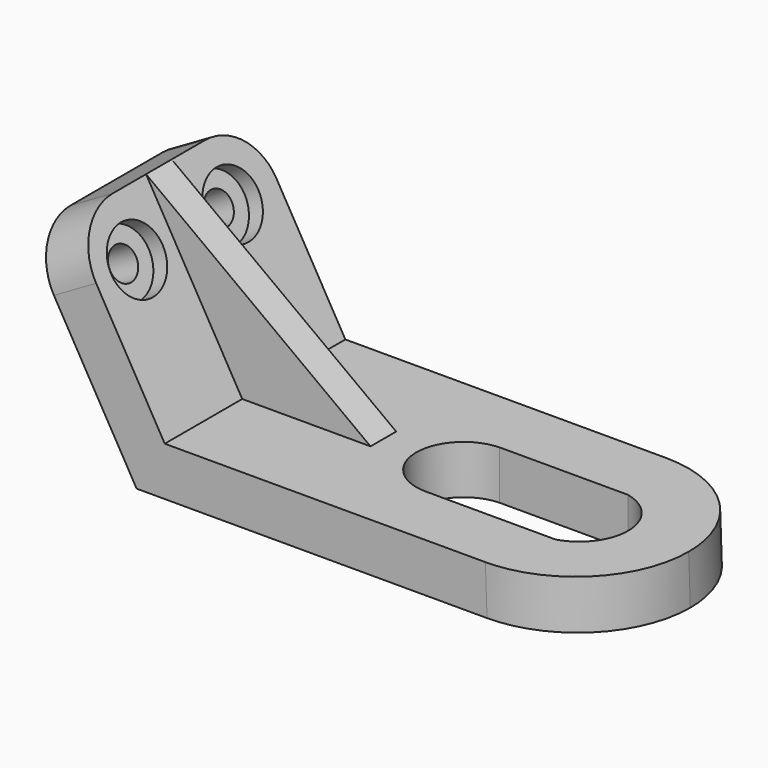
from build123d import *

# Parameters (mm, degrees)
F1_DEPTH  = 22.352
F2_DEPTH  = 3.175
F4_R      = 22.35199
F5_R      = 3.175
F6_DEPTH  = 25.4
F7_R      = 6.35
F7_R_2    = 3.175
F8_DEPTH  = 3.175
F9_R      = 10.922
F10_DEPTH = 25.4


# Not quite as in the source:
# - a fillet or chamfer is up to 0.001 mm smaller than in the source, because OpenCascade refuses the exact size


with BuildPart() as f1:
    # F0 (on Front) → F1 (new body, symmetric)
    with BuildSketch(Plane.XZ):
        Polygon((-3.9430456236, 0), (-29.3430456236, 0), (-48.3930456236, 32.9955678842), (-56.7519228209, 28.1695678842), (-34.9156304218, -9.652), (56.8391502193, -9.652), (56.5089543764, 0), align=None)
    extrude(amount=F1_DEPTH, both=True)

    # F0 (on Front) → F2 (join, symmetric)
    with BuildSketch(Plane.XZ):
        Polygon((-48.3930456236, 32.9955678842), (-29.3430456236, 0), (-3.9430456236, 0), align=None)
    extrude(amount=F2_DEPTH, both=True)

    # F4 (radius 22.352 in the source; OpenCascade refuses exactly that, so slightly less here)
    f4_edges = [f1.edges().sort_by_distance(p)[0] for p in [
        (56.674052, -22.352, -4.826),
        (56.674052, 22.352, -4.826),
    ]]
    fillet(f4_edges, radius=F4_R)

    # F5 (on face) → F6 (cut)
    with BuildSketch(Plane(origin=(-30.366161415, 0, -17.5319114672), x_dir=(0, -1, 0), z_dir=(-0.8660254038, 0, -0.5))):
        with Locations((-11.43, 41.8495228118)):
            Circle(F5_R)
        with Locations((12.2398376594, 41.8495228118)):
            Circle(F5_R)
    extrude(amount=-F6_DEPTH, mode=Mode.SUBTRACT)

    # F7 (on face) → F8 (cut)
    with BuildSketch(Plane(origin=(-22.0072842177, 0, -12.7059114672), x_dir=(0, 1, 0), z_dir=(0.8660254038, 0, 0.5))):
        with Locations((-12.2398376594, 41.8495228118)):
            Circle(F7_R)
        with Locations((-12.2398376594, 41.8495228118)):
            Circle(F7_R_2, mode=Mode.SUBTRACT)
        with Locations((11.43, 41.8495228118)):
            Circle(F7_R)
    extrude(amount=-F8_DEPTH, mode=Mode.SUBTRACT)

    # F9
    f9_edges = [f1.edges().sort_by_distance(p)[0] for p in [
        (-52.572484, 22.352, 30.582568),
        (-52.572484, -22.352, 30.582568),
    ]]
    fillet(f9_edges, radius=F9_R)

    # F3 (on face) → F10 (cut)
    with BuildSketch(Plane.XY):
        with BuildLine():
            Line((37.2716346684, 9.027880175), (11.8716346684, 9.027880175))
            ThreePointArc((11.8716346684, 9.027880175), (2.8515551479, -0.6319204795), (12.5113558024, -9.652))
            Line((12.5113558024, -9.652), (37.9113558024, -9.652))
            ThreePointArc((37.9113558024, -9.652), (44.825892917, -0.0643068731), (37.2716346684, 9.027880175))
        make_face()
    extrude(amount=-F10_DEPTH, mode=Mode.SUBTRACT)


solid = f1.part
